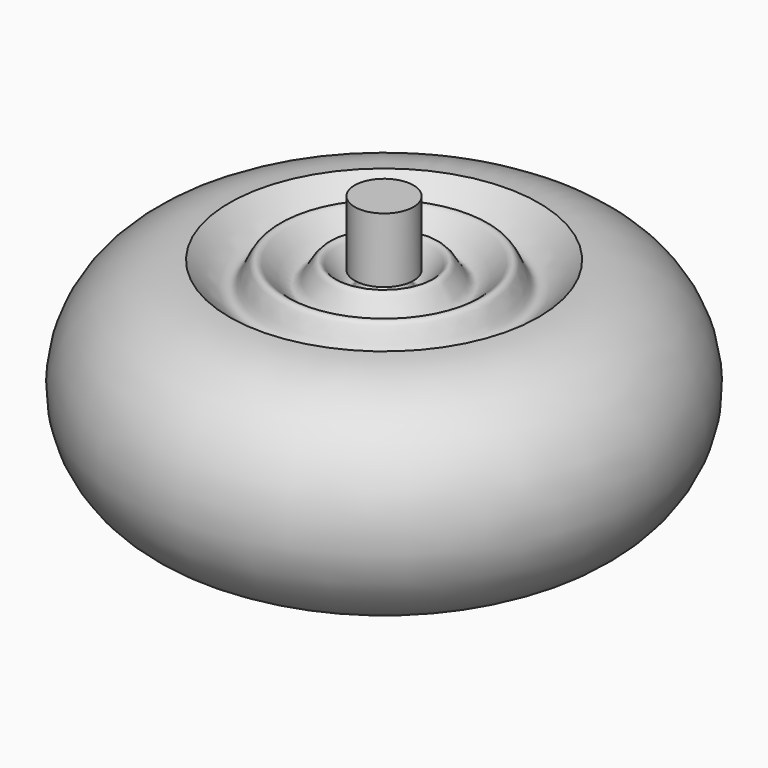
from build123d import *
from build123d import SkipClean  # not in build123d's __all__

# Parameters (mm, degrees)
F3_W      = 4.5995097607
F3_H      = 10.1451538503
F6_DEPTH  = 50.8
F8_DEPTH  = 50.8
F10_DEPTH = 50.8


with BuildPart() as f2:
    # F1 (on Front) → F2 (revolve)
    with BuildSketch(Plane.XZ):
        with BuildLine():
            add(Edge.make_bspline(
                [(0, 32.6588749886), (0, 21.7725833257), (0, 10.8862916629), (0, 0)],
                knots=[0, 0, 0, 0, 32.6588749886, 32.6588749886, 32.6588749886, 32.6588749886], degree=3))
            Line((0, 0), (24.2003984749, 0))
            ThreePointArc((24.2003984749, 0), (41.296819225, 17.09642075), (24.2003984749, 34.1928415))
            add(Edge.make_bspline(
                [(24.2003984749, 34.1928415), (21.9835400566, 31.7989092441), (17.9425179267, 27.4351063312), (16.3063234386, 37.5396964619), (10.7821231021, 27.2382084709), (8.1730019451, 37.782645751), (4.6367152438, 27.0449651457), (2.3802438015, 33.5777846299), (0.7144546351, 32.9346951596), (0, 32.6588749886)],
                knots=[0, 0, 0, 0, 0.1748700752, 0.3187636332, 0.4782745117, 0.6211924522, 0.7764606698, 0.9041242951, 1, 1, 1, 1], degree=3))
        make_face()
    revolve(axis=Axis((0, 0, -0.767044723), (0, 0, -1)))

    # F5 (on Front) → F6 (cut)
    with BuildSketch(Plane.XZ):
        Polygon((-9.4466600567, 23.0557732284), (-18.6564438045, 23.0557732284), (-13.4759396315, 17.4435619265), align=None)
        Polygon((13.2899954915, 17.8752690554), (17.17537269, 23.0557732284), (9.2640276998, 23.0236146599), align=None)
    extrude(amount=-F6_DEPTH, mode=Mode.SUBTRACT)

    # F7 (on Front) → F8 (cut)
    with BuildSketch(Plane.XZ):
        Polygon((0, 8.6227515712), (3.6529758945, 15.1497768238), (-5.0497250631, 15.1497768238), align=None)
    extrude(amount=-F8_DEPTH, mode=Mode.SUBTRACT)

    # F9 (on Front) → F10 (cut)
    with BuildSketch(Plane.XZ):
        with BuildLine():
            Line((6.6568879411, 6.7398734391), (-6.1107776128, 6.6040474921))
            ThreePointArc((-6.1107776128, 6.6040474921), (0.3428062193, 0.1153476514), (6.6568879411, 6.7398734391))
        make_face()
    with SkipClean():  # cleaning this boolean's faces spoils the solid; the shape is the same uncleaned
        extrude(amount=-F10_DEPTH, mode=Mode.SUBTRACT)


with BuildPart() as f4:
    # F3 (on Front) → F4 (revolve)
    with BuildSketch(Plane.XZ):
        with Locations((2.2997548804, 37.9109103233)):
            Rectangle(F3_W, F3_H)
    revolve(axis=Axis((0, 0, 37.9109103233), (0, 0, 1)))


solid = Compound([f2.part, f4.part])
